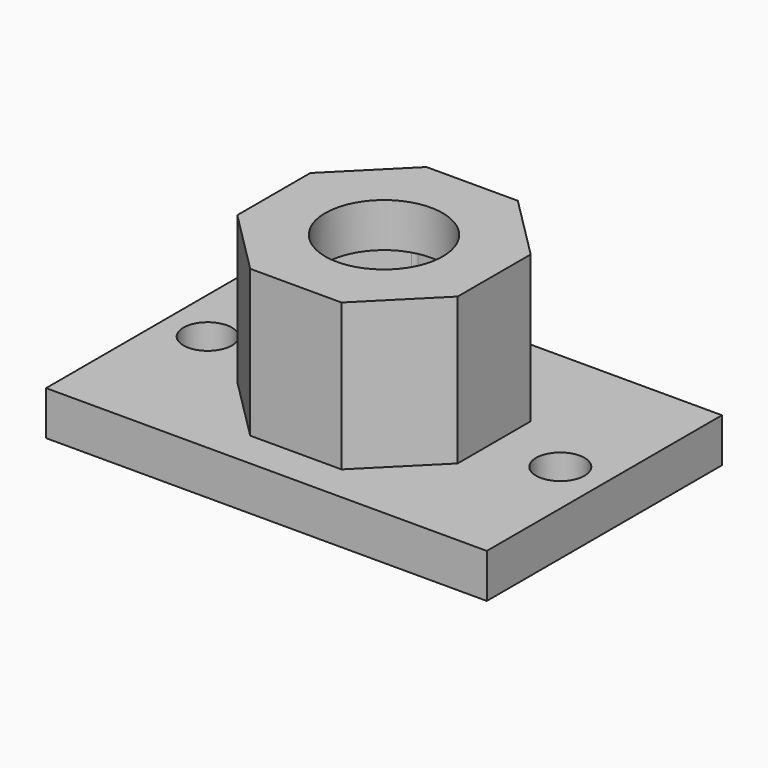
from build123d import *

# Parameters (mm, degrees)
F0_W         = 30
F0_H         = 3
F1_DEPTH     = 10
F3_DEPTH     = 10
F5_DEPTH     = 10
F7_D         = 8
F8_T1_DEPTH  = 10.517766953
F9_R         = 0.5
F10_T1_DEPTH = 10.517766953
F11_T1_DEPTH = 10.517766953
F12_T1_DEPTH = 10.517766953
F13_T1_DEPTH = 10.517766953
F14_T1_DEPTH = 10.517766953
F15_T1_DEPTH = 10.517766953
F17_D        = 3.3


# Not quite as in the source:
# - a fillet or chamfer that OpenCascade refuses, or shapes differently, is made with other operations: its cross-section is extruded or revolved along the edge and cut away or added
# - a feature names something its author has since deleted; it is built from what else it names


with BuildPart() as f1:
    # F0 (on Front) → F1 (new body, symmetric)
    with BuildSketch(Plane.XZ):
        Rectangle(F0_W, F0_H)
    extrude(amount=F1_DEPTH, both=True)

    # F2 (on face) → F3 (join)
    with BuildSketch(Plane.XY.offset(1.5)):
        Polygon((-3.1066017178, -7.5), (3.1066017178, -7.5), (7.5, -3.1066017178), (7.5, 3.1066017178), (3.1066017178, 7.5), (-3.1066017178, 7.5), (-7.5, 3.1066017178), (-7.5, -3.1066017178), align=None)
    extrude(amount=F3_DEPTH)

    # F4 (on face) → F5 (cut)
    with BuildSketch(Plane(origin=(0, 0, -1.5), x_dir=(1, 0, 0), z_dir=(0, 0, -1))):
        Polygon((-2.2781745931, -5.5), (2.2781745931, -5.5), (5.5, -2.2781745931), (5.5, 2.2781745931), (2.2781745931, 5.5), (-2.2781745931, 5.5), (-5.5, 2.2781745931), (-5.5, -2.2781745931), align=None)
    extrude(amount=-F5_DEPTH, mode=Mode.SUBTRACT)

    # F7 (through all)
    with Locations(Plane.XY.offset(11.5)):
        with Locations((0, 0)):
            Hole(F7_D / 2)

    # F8: fillet of radius 0.5 on 1 edges, made by hand

    # F8_s2 → F8_t1 (join)
    with BuildSketch(Plane.XY.offset(-1.5)):
        with BuildLine():
            add(Edge.make_bspline(
                [(2.4246212025, -5.3535533906), (2.2781745931, -5.5), (2.0710678119, -5.5)],
                knots=[0, 0, 0, 1, 1, 1], degree=2, weights=[1, 1, 1]))
            Line((2.0710678119, -5.5), (2.2781745931, -5.5))
            Line((2.2781745931, -5.5), (2.4246212025, -5.3535533906))
        make_face()
    extrude(amount=F8_T1_DEPTH)

    # F9
    f9_edges = [f1.edges().sort_by_distance(p)[0] for p in [
        (5.5, -2.278175, 3.5),
    ]]
    fillet(f9_edges, radius=F9_R)

    # F10: fillet of radius 0.5 on 1 edges, made by hand

    # F10_s2 → F10_t1 (join)
    with BuildSketch(Plane.XY.offset(-1.5)):
        with BuildLine():
            add(Edge.make_bspline(
                [(-2.0710678119, -5.5), (-2.2781745931, -5.5), (-2.4246212025, -5.3535533906)],
                knots=[0, 0, 0, 1, 1, 1], degree=2, weights=[1, 1, 1]))
            Line((-2.4246212025, -5.3535533906), (-2.2781745931, -5.5))
            Line((-2.2781745931, -5.5), (-2.0710678119, -5.5))
        make_face()
    extrude(amount=F10_T1_DEPTH)

    # F11: fillet of radius 0.5 on 1 edges, made by hand

    # F11_s2 → F11_t1 (join)
    with BuildSketch(Plane.XY.offset(-1.5)):
        with BuildLine():
            add(Edge.make_bspline(
                [(-5.3535533906, -2.4246212025), (-5.5, -2.2781745931), (-5.5, -2.0710678119)],
                knots=[0, 0, 0, 1, 1, 1], degree=2, weights=[1, 1, 1]))
            Line((-5.5, -2.0710678119), (-5.5, -2.2781745931))
            Line((-5.5, -2.2781745931), (-5.3535533906, -2.4246212025))
        make_face()
    extrude(amount=F11_T1_DEPTH)

    # F12: fillet of radius 0.5 on 1 edges, made by hand

    # F12_s2 → F12_t1 (join)
    with BuildSketch(Plane.XY.offset(-1.5)):
        with BuildLine():
            add(Edge.make_bspline(
                [(-5.3535533906, 2.4246212025), (-5.5, 2.2781745931), (-5.5, 2.0710678119)],
                knots=[0, 0, 0, 1, 1, 1], degree=2, weights=[1, 1, 1]))
            Line((-5.5, 2.0710678119), (-5.5, 2.2781745931))
            Line((-5.5, 2.2781745931), (-5.3535533906, 2.4246212025))
        make_face()
    extrude(amount=F12_T1_DEPTH)

    # F13: fillet of radius 0.5 on 1 edges, made by hand

    # F13_s2 → F13_t1 (join)
    with BuildSketch(Plane.XY.offset(-1.5)):
        with BuildLine():
            add(Edge.make_bspline(
                [(5.5, 2.0710678119), (5.5, 2.2781745931), (5.3535533906, 2.4246212025)],
                knots=[0, 0, 0, 1, 1, 1], degree=2, weights=[1, 1, 1]))
            Line((5.3535533906, 2.4246212025), (5.5, 2.2781745931))
            Line((5.5, 2.2781745931), (5.5, 2.0710678119))
        make_face()
    extrude(amount=F13_T1_DEPTH)

    # F14: fillet of radius 0.5 on 1 edges, made by hand

    # F14_s2 → F14_t1 (join)
    with BuildSketch(Plane.XY.offset(-1.5)):
        with BuildLine():
            add(Edge.make_bspline(
                [(2.4246212025, 5.3535533906), (2.2781745931, 5.5), (2.0710678119, 5.5)],
                knots=[0, 0, 0, 1, 1, 1], degree=2, weights=[1, 1, 1]))
            Line((2.0710678119, 5.5), (2.2781745931, 5.5))
            Line((2.2781745931, 5.5), (2.4246212025, 5.3535533906))
        make_face()
    extrude(amount=F14_T1_DEPTH)

    # F15: fillet of radius 0.5 on 1 edges, made by hand

    # F15_s2 → F15_t1 (join)
    with BuildSketch(Plane.XY.offset(-1.5)):
        with BuildLine():
            add(Edge.make_bspline(
                [(-2.0710678119, 5.5), (-2.2781745931, 5.5), (-2.4246212025, 5.3535533906)],
                knots=[0, 0, 0, 1, 1, 1], degree=2, weights=[1, 1, 1]))
            Line((-2.4246212025, 5.3535533906), (-2.2781745931, 5.5))
            Line((-2.2781745931, 5.5), (-2.0710678119, 5.5))
        make_face()
    extrude(amount=F15_T1_DEPTH)

    # F17 (through all)
    with Locations(Plane.XY.offset(1.5)):
        with Locations((-12, 0), (12, 0)):
            Hole(F17_D / 2)


solid = f1.part
